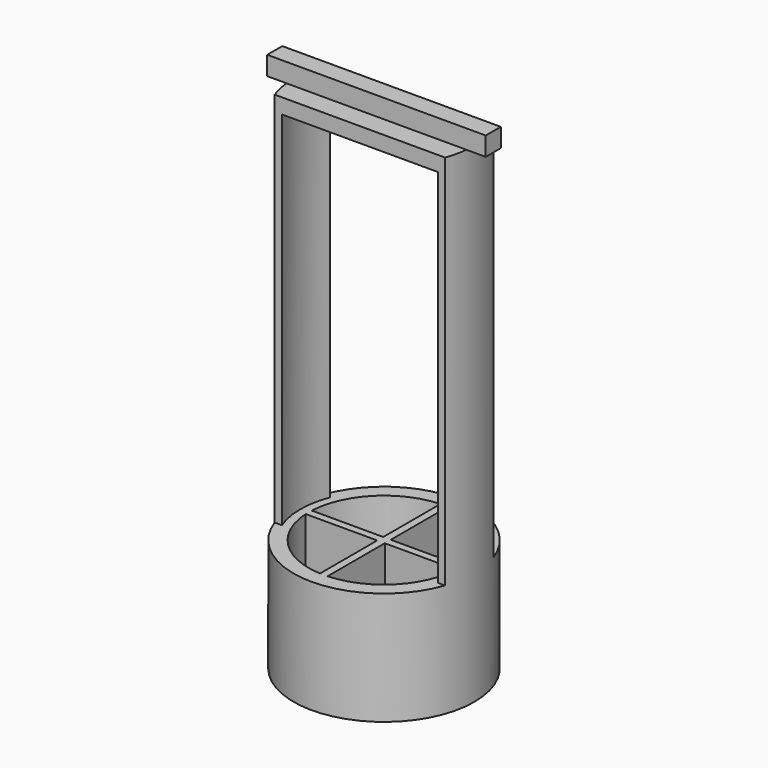
from build123d import *

# Parameters (mm, degrees)
F0_R      = 12
F1_DEPTH  = 15
F3_DEPTH  = 15.001
F4_R      = 12
F4_R_2    = 11.1
F5_DEPTH  = 50
F7_DEPTH  = 50
F8_W      = 22.627416998
F8_H      = 8
F9_DEPTH  = 2
F10_W     = 29
F10_H     = 2.5
F11_DEPTH = 2.5


with BuildPart() as f1:
    # F0 (on Top) → F1 (new body)
    with BuildSketch(Plane.XY):
        Circle(F0_R)
    extrude(amount=F1_DEPTH)

    # F2 (on face) → F3 (cut, through all)
    with BuildSketch(Plane.XY.offset(15)):
        with BuildLine():
            Line((-0.5, 0.5), (-0.5, 9.9874921777))
            ThreePointArc((-0.5, 9.9874921777), (-7.0710678119, 7.0710678119), (-9.9874921777, 0.5))
            Line((-9.9874921777, 0.5), (-0.5, 0.5))
        make_face()
        with BuildLine():
            Line((0.5, 0.5), (9.9874921777, 0.5))
            ThreePointArc((9.9874921777, 0.5), (7.0710678119, 7.0710678119), (0.5, 9.9874921777))
            Line((0.5, 9.9874921777), (0.5, 0.5))
        make_face()
        with BuildLine():
            ThreePointArc((0.5, -9.9874921777), (7.0710678119, -7.0710678119), (9.9874921777, -0.5))
            Line((9.9874921777, -0.5), (0.5, -0.5))
            Line((0.5, -0.5), (0.5, -9.9874921777))
        make_face()
        with BuildLine():
            ThreePointArc((-9.9874921777, -0.5), (-7.0710678119, -7.0710678119), (-0.5, -9.9874921777))
            Line((-0.5, -9.9874921777), (-0.5, -0.5))
            Line((-0.5, -0.5), (-9.9874921777, -0.5))
        make_face()
    extrude(amount=-F3_DEPTH, mode=Mode.SUBTRACT)

    # F4 (on face) → F5 (join)
    with BuildSketch(Plane.XY.offset(15)):
        Circle(F4_R)
        Circle(F4_R_2, mode=Mode.SUBTRACT)
    extrude(amount=F5_DEPTH)

    # F6 (on face) → F7 (cut)
    with BuildSketch(Plane.XY.offset(65)):
        with BuildLine():
            Line((14.9746745975, -4), (14.8116537966, -4))
            Line((14.8116537966, -4), (11.313708499, -4))
            ThreePointArc((11.313708499, -4), (0, -12), (-11.313708499, -4))
            Line((-11.313708499, -4), (-14.8116537966, -4))
            Line((-14.8116537966, -4), (-14.8116537966, -14.8480758196))
            Line((-14.8116537966, -14.8480758196), (14.9746745975, -14.8480758196))
            Line((14.9746745975, -14.8480758196), (14.9746745975, -4))
        make_face()
        with BuildLine():
            Line((11.313708499, -4), (14.8116537966, -4))
            Line((14.8116537966, -4), (14.8116537966, 4))
            Line((14.8116537966, 4), (11.313708499, 4))
            ThreePointArc((11.313708499, 4), (11.8271827158, 2.0292237447), (12, 0))
            ThreePointArc((12, 0), (11.8271827158, -2.0292237447), (11.313708499, -4))
        make_face()
        with BuildLine():
            ThreePointArc((-11.313708499, -4), (0, -12), (11.313708499, -4))
            Line((11.313708499, -4), (10.3542261903, -4))
            ThreePointArc((10.3542261903, -4), (0, -11.1), (-10.3542261903, -4))
            Line((-10.3542261903, -4), (-11.313708499, -4))
        make_face()
        with BuildLine():
            Line((11.313708499, 4), (14.8116537966, 4))
            Line((14.8116537966, 4), (15.4569065875, 4))
            Line((15.4569065875, 4), (15.4569065875, 13.0318450025))
            Line((15.4569065875, 13.0318450025), (-14.8116537966, 13.0318450025))
            Line((-14.8116537966, 13.0318450025), (-14.8116537966, 4))
            Line((-14.8116537966, 4), (-11.313708499, 4))
            ThreePointArc((-11.313708499, 4), (0, 12), (11.313708499, 4))
        make_face()
        with BuildLine():
            Line((-10.3542261903, -4), (10.3542261903, -4))
            ThreePointArc((10.3542261903, -4), (10.9119638634, -2.0344642154), (11.1, 0))
            ThreePointArc((11.1, 0), (10.9119638634, 2.0344642154), (10.3542261903, 4))
            Line((10.3542261903, 4), (-10.3542261903, 4))
            ThreePointArc((-10.3542261903, 4), (-11.1, 0), (-10.3542261903, -4))
        make_face()
        with BuildLine():
            Line((10.3542261903, 4), (11.313708499, 4))
            ThreePointArc((11.313708499, 4), (0, 12), (-11.313708499, 4))
            Line((-11.313708499, 4), (-10.3542261903, 4))
            ThreePointArc((-10.3542261903, 4), (0, 11.1), (10.3542261903, 4))
        make_face()
    extrude(amount=-F7_DEPTH, mode=Mode.SUBTRACT)

    # F8 (on face) → F9 (join)
    with BuildSketch(Plane.XY.offset(65)):
        Rectangle(F8_W, F8_H)
    extrude(amount=-F9_DEPTH)

    # F10 (on face) → F11 (join)
    with BuildSketch(Plane.XY.offset(65)):
        Rectangle(F10_W, F10_H)
    extrude(amount=F11_DEPTH)


solid = f1.part
